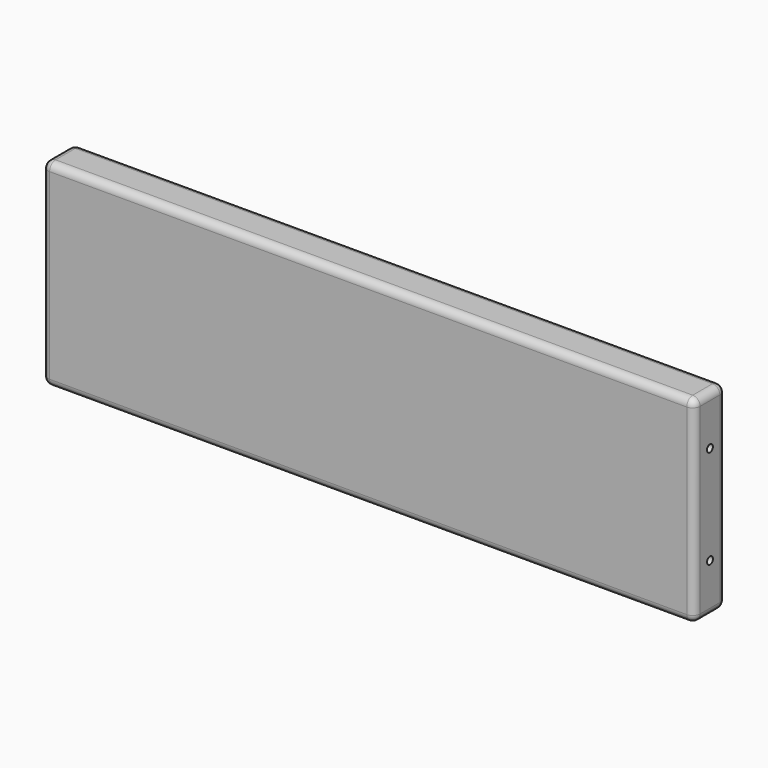
from build123d import *

# Parameters (mm, degrees)
F0_W         = 335.28
F0_H         = 101.6
F1_DEPTH     = 10.16
F2_R         = 3.81
F4_D         = 3.81
F4_DEPTH     = 12.7
F4_TIP       = 1.1446394792
F5_D         = 3.81
F5_DEPTH     = 12.7
F5_TIP       = 1.1446394792
F6_T1_DEPTH  = 12.7
F6_S5_W      = 3.81
F6_S5_H      = 3.81
F6_T6_DEPTH  = 3.81
F6_S11_W     = 3.81
F6_S11_H     = 3.81
F6_T12_DEPTH = 3.81
F8_D         = 3.81
F8_DEPTH     = 12.7
F8_TIP       = 1.1446394792
F9_D         = 3.81
F9_DEPTH     = 12.7
F9_TIP       = 1.1446394792


# Not quite as in the source:
# - a fillet or chamfer that OpenCascade refuses, or shapes differently, is made with other operations: its cross-section is extruded or revolved along the edge and cut away or added


with BuildPart() as f1:
    # F0 (on Front) → F1 (new body, symmetric)
    with BuildSketch(Plane.XZ):
        with Locations((-42.0896737862, 32.6920958787)):
            Rectangle(F0_W, F0_H)
    extrude(amount=F1_DEPTH, both=True)

    # F2
    f2_edges = [f1.edges().sort_by_distance(p)[0] for p in [
        (-42.089674, -10.16, 83.492096),
        (-209.729674, -10.16, 32.692096),
        (-42.089674, -10.16, -18.107904),
        (125.550326, -10.16, 32.692096),
        (-42.089674, 10.16, -18.107904),
        (-42.089674, 10.16, 83.492096),
        (-209.729674, 10.16, 32.692096),
        (125.550326, 10.16, 32.692096),
        (125.550326, 0, 83.492096),
        (125.550326, 0, -18.107904),
        (-209.729674, 0, 83.492096),
    ]]
    fillet(f2_edges, radius=F2_R)

    # F4
    with Locations(Plane.YZ.offset(125.5503262138)):
        with Locations((0, 58.0920958787)):
            Hole(F4_D / 2, depth=F4_DEPTH)
            with Locations((0, 0, -(F4_DEPTH + F4_TIP / 2))):  # 118° drill point
                Cone(0, F4_D / 2, F4_TIP, mode=Mode.SUBTRACT)

    # F5
    with Locations(Plane.YZ.offset(125.5503262138)):
        with Locations((0, 7.2920958787)):
            Hole(F5_D / 2, depth=F5_DEPTH)
            with Locations((0, 0, -(F5_DEPTH + F5_TIP / 2))):  # 118° drill point
                Cone(0, F5_D / 2, F5_TIP, mode=Mode.SUBTRACT)

    # F6: fillet of radius 3.81 on 1 edges, made by hand

    # F6_s2 → F6_t1 (cut)
    with BuildSketch(Plane.XZ.offset(-6.35)):
        with BuildLine():
            ThreePointArc((-209.7296737862, -14.2979041213), (-208.6137506225, -16.9919809576), (-205.9196737862, -18.1079041213))
            Line((-205.9196737862, -18.1079041213), (-209.7296737862, -18.1079041213))
            Line((-209.7296737862, -18.1079041213), (-209.7296737862, -14.2979041213))
        make_face()
    extrude(amount=F6_T1_DEPTH, mode=Mode.SUBTRACT)


with BuildPart() as f6_tool4:
    # F6_s5 → F6_t6 (new body)
    with BuildSketch(Plane.YZ.offset(-205.9196737862)):
        with Locations((8.255, -16.2029041213)):
            Rectangle(F6_S5_W, F6_S5_H)
    extrude(amount=-F6_T6_DEPTH)

    # F6_s7 → F6_t8 (revolve, cut)
    with BuildSketch(Plane(origin=(-205.9196737862, 6.35, -14.2979041213), x_dir=(0, -0.7071067812, 0.7071067812), z_dir=(0, -0.7071067812, -0.7071067812))):
        with BuildLine():
            ThreePointArc((0, -3.81), (3.81, 0), (0, 3.81))
            Line((0, 3.81), (0, -3.81))
        make_face()
    revolve(axis=Axis((-205.9196737862, 6.35, -14.2979041213), (-1, 0, 0)), mode=Mode.SUBTRACT)


with BuildPart() as f1_1:
    add(f1.part)

    # F6_t3: cut F6_tool4
    add(f6_tool4.part, mode=Mode.SUBTRACT)


with BuildPart() as f6_tool10:
    # F6_s11 → F6_t12 (new body)
    with BuildSketch(Plane.YZ.offset(-205.9196737862)):
        with Locations((-8.255, -16.2029041213)):
            Rectangle(F6_S11_W, F6_S11_H)
    extrude(amount=-F6_T12_DEPTH)

    # F6_s13 → F6_t14 (revolve, cut)
    with BuildSketch(Plane(origin=(-205.9196737862, -6.35, -14.2979041213), x_dir=(0, 0.7071067812, 0.7071067812), z_dir=(0, -0.7071067812, 0.7071067812))):
        with BuildLine():
            ThreePointArc((0, -3.81), (3.81, 0), (0, 3.81))
            Line((0, 3.81), (0, -3.81))
        make_face()
    revolve(axis=Axis((-205.9196737862, -6.35, -14.2979041213), (-1, 0, 0)), mode=Mode.SUBTRACT)


with BuildPart() as f1_2:
    add(f1_1.part)

    # F6_t9: cut F6_tool10
    add(f6_tool10.part, mode=Mode.SUBTRACT)

    # F8
    with Locations(Plane(origin=(-209.7296737862, 0, 0), x_dir=(0, -1, 0), z_dir=(-1, 0, 0))):
        with Locations((0, 58.0920958787)):
            Hole(F8_D / 2, depth=F8_DEPTH)
            with Locations((0, 0, -(F8_DEPTH + F8_TIP / 2))):  # 118° drill point
                Cone(0, F8_D / 2, F8_TIP, mode=Mode.SUBTRACT)

    # F9
    with Locations(Plane(origin=(-209.7296737862, 0, 0), x_dir=(0, -1, 0), z_dir=(-1, 0, 0))):
        with Locations((0, 7.2920958787)):
            Hole(F9_D / 2, depth=F9_DEPTH)
            with Locations((0, 0, -(F9_DEPTH + F9_TIP / 2))):  # 118° drill point
                Cone(0, F9_D / 2, F9_TIP, mode=Mode.SUBTRACT)


solid = f1_2.part
